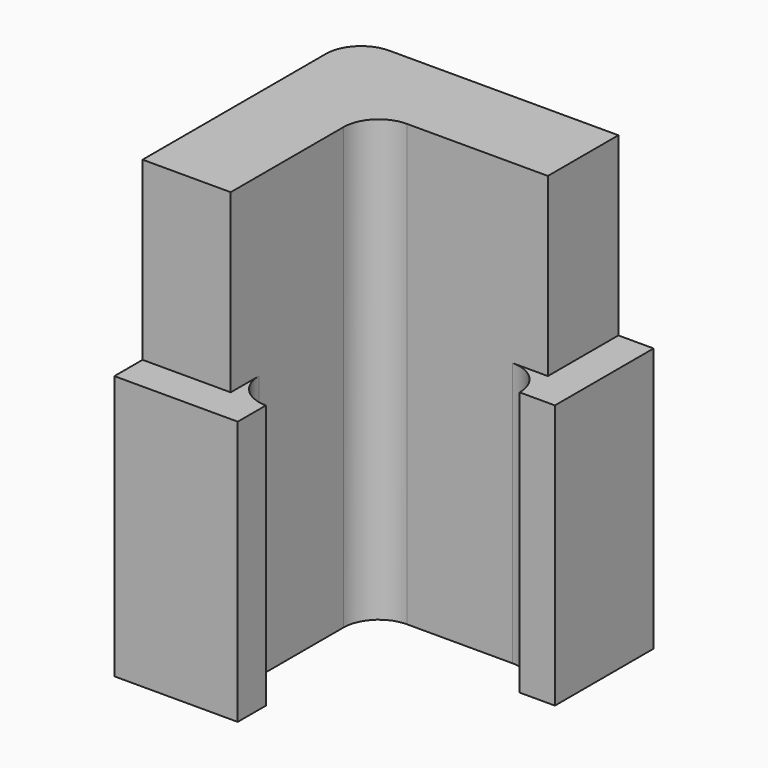
from build123d import *

# Parameters (mm, degrees)
F1_DEPTH = 25
F2_R     = 2
F3_DEPTH = 15
F4_R     = 1.99999


# Not quite as in the source:
# - a fillet or chamfer is up to 0.001 mm smaller than in the source, because OpenCascade refuses the exact size


with BuildPart() as f1:
    # F0 (on Top) → F1 (new body)
    with BuildSketch(Plane.XY):
        Polygon((15, 0), (0, 0), (0, -15), (5, -15), (5, -5), (15, -5), align=None)
    extrude(amount=F1_DEPTH)

    # F2
    f2_edges = [f1.edges().sort_by_distance(p)[0] for p in [
        (5, -5, 12.5),
        (0, 0, 12.5),
    ]]
    fillet(f2_edges, radius=F2_R)

    # F0 (on Top) → F3 (join)
    with BuildSketch(Plane.XY):
        Polygon((5, -15), (0, -15), (0, -17), (7, -17), (7, -15), align=None)
        Polygon((17, 0), (15, 0), (15, -5), (15, -7), (17, -7), align=None)
    extrude(amount=F3_DEPTH)

    # F4 (radius 2 in the source; OpenCascade refuses exactly that, so slightly less here)
    f4_edges = [f1.edges().sort_by_distance(p)[0] for p in [
        (5, -15, 7.5),
        (15, -5, 7.5),
    ]]
    fillet(f4_edges, radius=F4_R)


solid = f1.part
